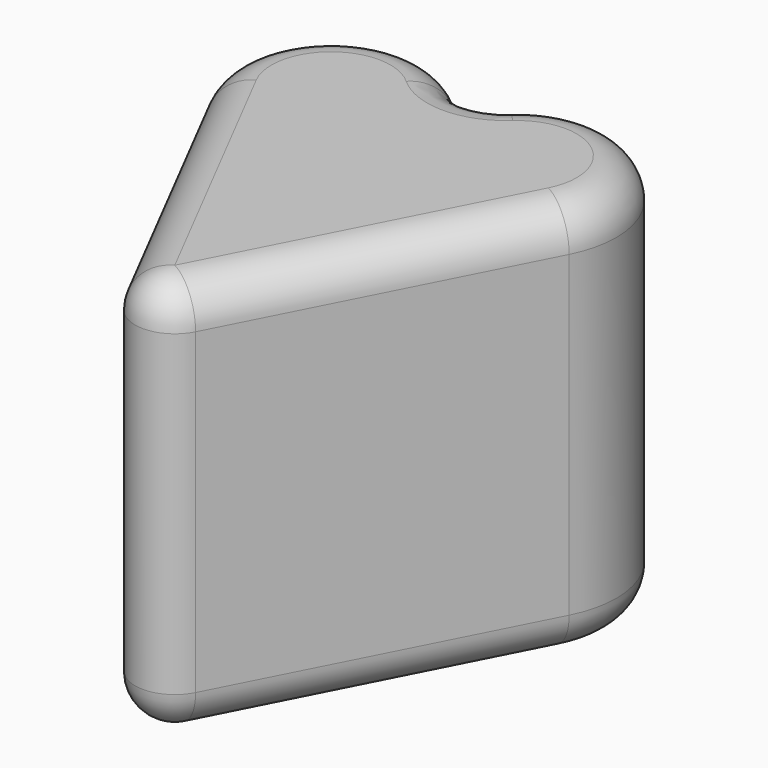
from build123d import *

# Parameters (mm, degrees)
F1_DEPTH = 20
F2_F1_R  = 2
F2_F2_R  = 2
F2_F3_R  = 2


with BuildPart() as f1:
    # F0 (on Top) → F1 (new body)
    with BuildSketch(Plane.XY):
        with BuildLine():
            ThreePointArc((0, 3.4753886408), (-6.702786735, 6.3139324677), (-9.1361551027, -0.5463444553))
            Line((-9.1361551027, -0.5463444553), (0, -18.3376532868))
            Line((0, -18.3376532868), (9.1361551027, -0.5463444553))
            ThreePointArc((9.1361551027, -0.5463444553), (6.702786735, 6.3139324677), (0, 3.4753886408))
        make_face()
        with BuildLine():
            ThreePointArc((0, 0), (-0.3116721052, 1.7376943204), (0, 3.4753886408))
            ThreePointArc((0, 3.4753886408), (0.3116721052, 1.7376943204), (0, 0))
        make_face(mode=Mode.SUBTRACT)
        with BuildLine():
            ThreePointArc((0, 0), (0.3116721052, 1.7376943204), (0, 3.4753886408))
            ThreePointArc((0, 3.4753886408), (-0.3116721052, 1.7376943204), (0, 0))
        make_face()
    extrude(amount=F1_DEPTH)

    # F2: fillet of radius 2 on 7 edges, made by hand

    # F2_f1
    f2_f1_edges = [f1.edges().sort_by_distance(p)[0] for p in [
        (0, 3.4753886408, 10),
    ]]
    fillet(f2_f1_edges, radius=F2_F1_R)

    # F2_f2
    f2_f2_edges = [f1.edges().sort_by_distance(p)[0] for p in [
        (0, -18.3376532868, 10),
    ]]
    fillet(f2_f2_edges, radius=F2_F2_R)

    # F2_f3
    f2_f3_edges = [f1.edges().sort_by_distance(p)[0] for p in [
        (7.7367258426, 5.7009341506, 0),
        (7.7367258426, 5.7009341506, 20),
        (5.4576429929, -7.7097019344, 0),
        (5.4576429929, -7.7097019344, 20),
        (0, -15.9594439033, 20),
        (0, -15.9594439033, 0),
        (1e-10, 4.9357306327, 20),
        (1e-10, 4.9357306327, 0),
    ]]
    fillet(f2_f3_edges, radius=F2_F3_R)


solid = f1.part
